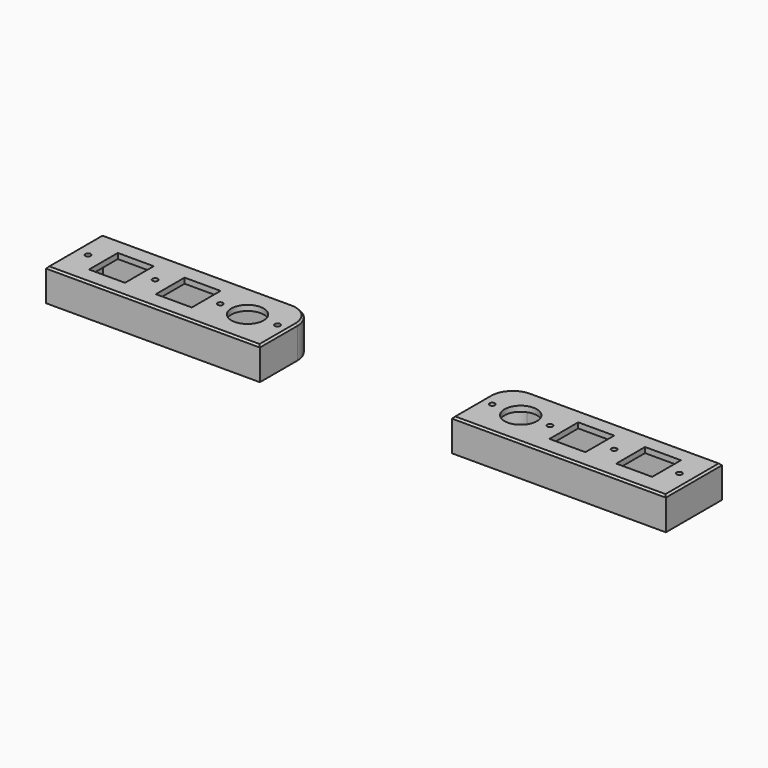
from build123d import *

# Parameters (mm, degrees)
F1_DEPTH      = 5
F1_DEPTH_BACK = 10
F2_T          = 3
F2_2_T        = 3
F4_W          = 20
F4_H          = 20
F4_H_2        = 20.0000037253
F4_R          = 9
F5_DEPTH      = 50
F8_D          = 3
F8_DEPTH      = 40
F8_TIP        = 0.9012909285
F8_2_D        = 3
F8_2_DEPTH    = 40
F8_2_TIP      = 0.9012909285
F9_SIZE       = 1
F9_2_SIZE     = 1


with BuildPart() as f1:
    # F0 (on Top) → F1 (new body, two sides)
    with BuildSketch(Plane.XY) as f1_sk:
        with BuildLine():
            Line((169.1123094261, 78.8974409995), (66.1123094261, 78.8974409995))
            ThreePointArc((66.1123094261, 78.8974409995), (59.0412416142, 75.9685088113), (56.1123094261, 68.8974409995))
            Line((56.1123094261, 68.8974409995), (56.1123094261, 45.8974409995))
            Line((56.1123094261, 45.8974409995), (169.1123094261, 45.8974409995))
            Line((169.1123094261, 45.8974409995), (169.1123094261, 78.8974409995))
        make_face()
    extrude(amount=F1_DEPTH)
    extrude(f1_sk.sketch, amount=-F1_DEPTH_BACK)

    # F2
    f2_openings = [f1.faces().sort_by_distance(p)[0] for p in [
        (112.926417, 62.314864, -10),
    ]]
    offset(amount=F2_T, openings=f2_openings, kind=Kind.INTERSECTION)


with BuildPart() as f1b:
    # F0 (on Top) → F1, piece 2 (new body, two sides)
    with BuildSketch(Plane.XY) as f1_2_sk:
        with BuildLine():
            Line((-66.9198182523, 78.9953285099), (-169.9198182523, 78.9953285099))
            Line((-169.9198182523, 78.9953285099), (-169.9198182523, 45.9953285099))
            Line((-169.9198182523, 45.9953285099), (-56.9198182523, 45.9953285099))
            Line((-56.9198182523, 45.9953285099), (-56.9198182523, 68.9953285099))
            ThreePointArc((-56.9198182523, 68.9953285099), (-59.8487504405, 76.0663963218), (-66.9198182523, 78.9953285099))
        make_face()
    extrude(amount=F1_DEPTH)
    extrude(f1_2_sk.sketch, amount=-F1_DEPTH_BACK)

    # F2#2
    f2_2_openings = [f1b.faces().sort_by_distance(p)[0] for p in [
        (-113.733926, 62.412751, -10),
    ]]
    offset(amount=F2_2_T, openings=f2_2_openings, kind=Kind.INTERSECTION)


with BuildPart() as f5_tool:
    # F4 (on offset) → F5 (new body)
    with BuildSketch(Plane.XY.offset(33)):
        with Locations((-146.575255096, 62.4660721421)):
            Rectangle(F4_W, F4_H)
        with Locations((-109.3974763155, 62.4660702795)):
            Rectangle(F4_W, F4_H_2)
        with Locations((-76.3929139701, 62.4939369033)):
            Circle(F4_R)
        with Locations((75.5820007977, 62.6008242587)):
            Circle(F4_R)
        with Locations((109.2696897686, 62.9745572805)):
            Rectangle(F4_W, F4_H)
        with Locations((146.447468549, 62.9745554179)):
            Rectangle(F4_W, F4_H_2)
    extrude(amount=-F5_DEPTH)


with BuildPart() as f1_1:
    add(f1.part)

    # F5: cut by f5_tool
    add(f5_tool.part, mode=Mode.SUBTRACT)

    # F8
    with Locations(Plane.XY.offset(8)):
        with Locations((-128.1331330538, 62.8871805966), (163.6322605932, 62.8871805966), (127.36319817, 62.8871805966), (-165.489256382, 62.8871805966), (91.6408523917, 62.8871805966), (59.4655014575, 62.8871805966), (-91.8687133804, 62.8871805966), (-59.9663094311, 62.8871805966)):
            Hole(F8_D / 2, depth=F8_DEPTH)
            with Locations((0, 0, -(F8_DEPTH + F8_TIP / 2))):  # 118° drill point
                Cone(0, F8_D / 2, F8_TIP, mode=Mode.SUBTRACT)

    # F9
    f9_edges = [f1_1.edges().sort_by_distance(p)[0] for p in [
        (112.612309, 42.897441, 8),
        (172.112309, 62.397441, 8),
        (119.112309, 81.897441, 8),
        (56.919921, 78.089829, 8),
        (53.112309, 55.897441, 8),
    ]]
    chamfer(f9_edges, length=F9_SIZE)


with BuildPart() as f1b_1:
    add(f1b.part)

    # F5: cut by f5_tool
    add(f5_tool.part, mode=Mode.SUBTRACT)

    # F8#2
    with Locations(Plane.XY.offset(8)):
        with Locations((-128.1331330538, 62.8871805966), (163.6322605932, 62.8871805966), (127.36319817, 62.8871805966), (-165.489256382, 62.8871805966), (91.6408523917, 62.8871805966), (59.4655014575, 62.8871805966), (-91.8687133804, 62.8871805966), (-59.9663094311, 62.8871805966)):
            Hole(F8_2_D / 2, depth=F8_2_DEPTH)
            with Locations((0, 0, -(F8_2_DEPTH + F8_2_TIP / 2))):  # 118° drill point
                Cone(0, F8_2_D / 2, F8_2_TIP, mode=Mode.SUBTRACT)

    # F9#2
    f9_2_edges = [f1b_1.edges().sort_by_distance(p)[0] for p in [
        (-53.919818, 55.995329, 8),
        (-57.72743, 78.187717, 8),
        (-119.919818, 81.995329, 8),
        (-172.919818, 62.495329, 8),
        (-113.419818, 42.995329, 8),
    ]]
    chamfer(f9_2_edges, length=F9_2_SIZE)


solid = Compound([f1_1.part, f1b_1.part])
